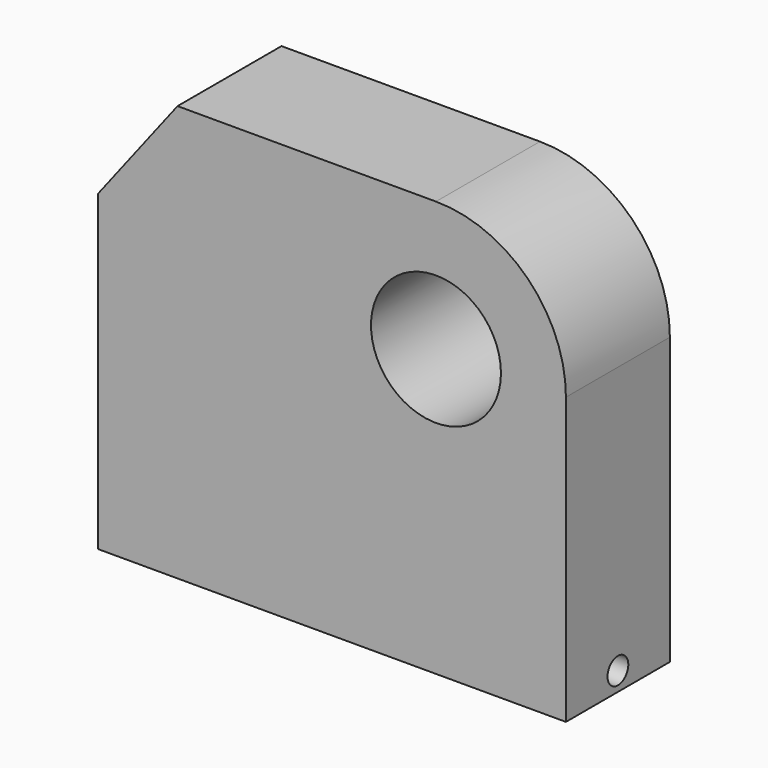
from build123d import *

# Parameters (mm, degrees)
F0_R     = 12.5
F1_DEPTH = 12.5
F2_DEPTH = 12.501
F3_DEPTH = 12.5
F4_R     = 1.5
F5_DEPTH = 25
F6_R     = 2.5
F7_DEPTH = 90.001


# Not quite as in the source:
# - a feature names something its author has since deleted; it is built from what else it names


with BuildPart() as f1:
    # F0 (on Front) → F1 (new body, symmetric)
    with BuildSketch(Plane.XZ):
        Polygon((25.6665702909, 80), (15.280091039, 80), (0, 60.2131655427), (0, 40.0504879653), align=None)
        with BuildLine():
            Line((65, 80), (25.6665702909, 80))
            Line((25.6665702909, 80), (0, 40.0504879653))
            Line((0, 40.0504879653), (0, 0))
            Line((0, 0), (90, 0))
            Line((90, 0), (90, 55))
            ThreePointArc((90, 55), (82.6776695297, 72.6776695297), (65, 80))
        make_face()
        with Locations((65, 55)):
            Circle(F0_R, mode=Mode.SUBTRACT)
    extrude(amount=F1_DEPTH, both=True)

    # F0 (on Front) → F2 (cut, through all)
    with BuildSketch(Plane.XZ):
        Polygon((25.6665702909, 80), (15.280091039, 80), (0, 60.2131655427), (0, 40.0504879653), align=None)
        with BuildLine():
            Line((65, 80), (25.6665702909, 80))
            Line((25.6665702909, 80), (0, 40.0504879653))
            Line((0, 40.0504879653), (0, 0))
            Line((0, 0), (90, 0))
            Line((90, 0), (90, 55))
            ThreePointArc((90, 55), (82.6776695297, 72.6776695297), (65, 80))
        make_face()
        with Locations((65, 55)):
            Circle(F0_R, mode=Mode.SUBTRACT)
    extrude(amount=-F2_DEPTH, mode=Mode.SUBTRACT)

    # F0 (on Front) → F3 (join, symmetric)
    with BuildSketch(Plane.XZ):
        Polygon((25.6665702909, 80), (15.280091039, 80), (0, 60.2131655427), (0, 40.0504879653), align=None)
        with BuildLine():
            Line((65, 80), (25.6665702909, 80))
            Line((25.6665702909, 80), (0, 40.0504879653))
            Line((0, 40.0504879653), (0, 0))
            Line((0, 0), (90, 0))
            Line((90, 0), (90, 55))
            ThreePointArc((90, 55), (82.6776695297, 72.6776695297), (65, 80))
        make_face()
        with Locations((65, 55)):
            Circle(F0_R, mode=Mode.SUBTRACT)
    extrude(amount=F3_DEPTH, both=True)

    # F4 (on Right) → F5 (cut)
    with BuildSketch(Plane.YZ):
        with Locations((0, 22)):
            Circle(F4_R)
        with Locations((0, 42)):
            Circle(F4_R)
    extrude(amount=F5_DEPTH, mode=Mode.SUBTRACT)

    # F6 (on face) → F7 (cut, through all)
    with BuildSketch(Plane.YZ.offset(90)):
        with Locations((0, 3.611382097)):
            Circle(F6_R)
    extrude(amount=-F7_DEPTH, mode=Mode.SUBTRACT)


solid = f1.part
